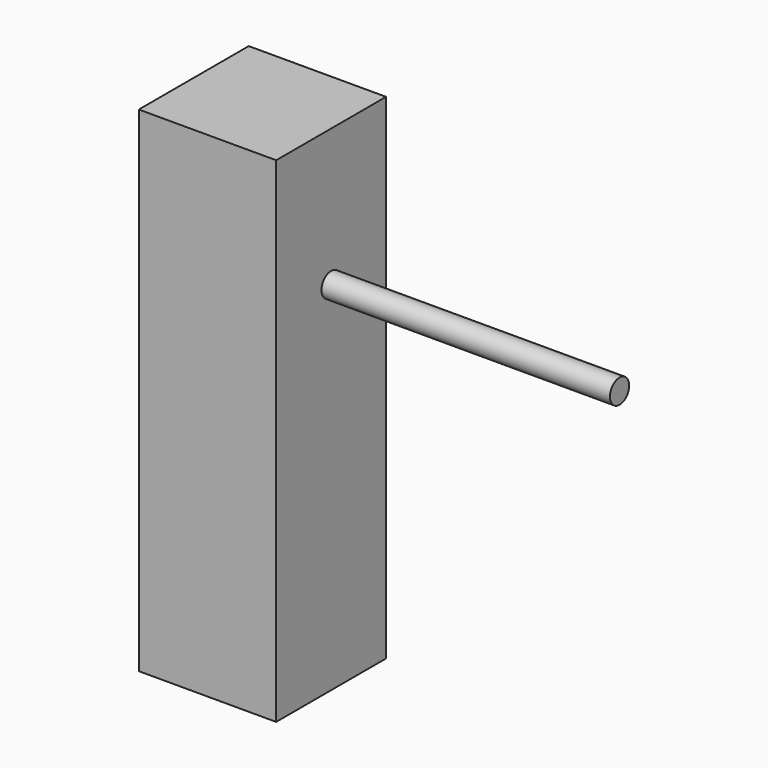
from build123d import *

# Parameters (mm, degrees)
F0_W     = 127
F0_H     = 127
F1_DEPTH = 457.2
F2_R     = 11.1125
F3_DEPTH = 266.7


# Not quite as in the source:
# - a feature names something its author has since deleted; it is built from what else it names


with BuildPart() as f1:
    # F0 (on Top) → F1 (new body)
    with BuildSketch(Plane.XY):
        with Locations((63.5, -63.5)):
            Rectangle(F0_W, F0_H)
    extrude(amount=F1_DEPTH)

    # F2 (on face) → F3 (join)
    with BuildSketch(Plane.YZ.offset(127)):
        with Locations((-63.5, 330.2)):
            Circle(F2_R)
    extrude(amount=F3_DEPTH)


solid = f1.part
